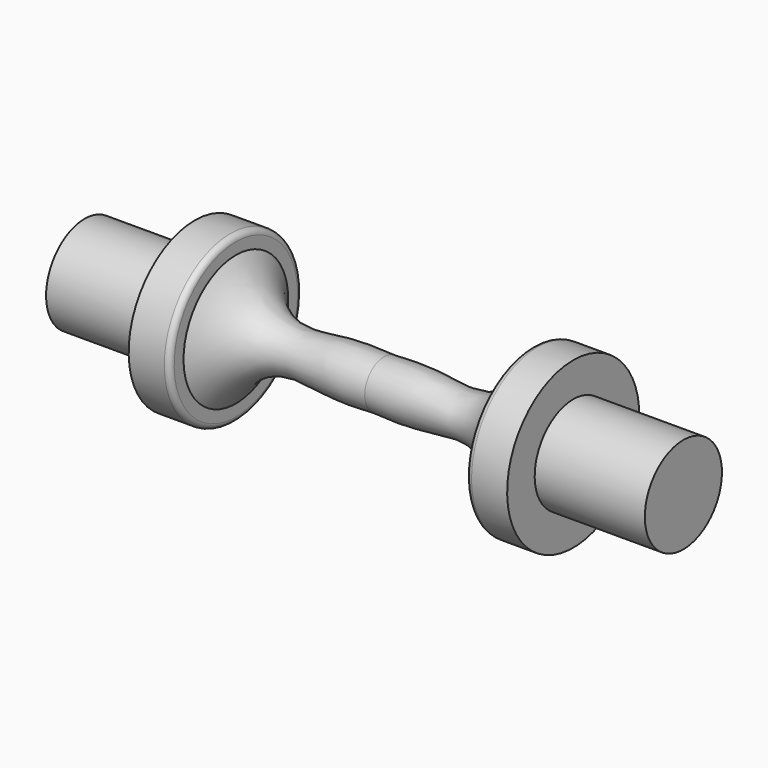
from build123d import *


with BuildPart() as f1:
    # F0 (on Front) → F1 (revolve)
    with BuildSketch(Plane.XZ):
        with BuildLine():
            Line((0, 8.75), (0, 0))
            Line((0, 0), (108.719505762, 0))
            Line((108.719505762, 0), (108.719505762, 17.5))
            Line((108.719505762, 17.5), (68.719505762, 17.5))
            Line((68.719505762, 17.5), (68.719505762, 30))
            Line((68.719505762, 30), (55.7926830174, 30))
            ThreePointArc((55.7926830174, 30), (54.3784694551, 29.4142135624), (53.7926830174, 28))
            Line((53.7926830174, 28), (53.7926830174, 23.75))
            add(Edge.make_bspline(
                [(0, 8.75), (5.0406153604, 9.0258980354), (16.3424850669, 9.5343195461), (38.0075656916, 5.0292358393), (49.6364947054, 17.2036020787), (53.7926830174, 23.75)],
                knots=[0, 0, 0, 0, 0.3026453885, 0.6427893554, 1, 1, 1, 1], degree=3))
        make_face()
    revolve(axis=Axis((54.359752881, 0, 0), (-1, 0, 0)))

    # F2: F1 across face


with BuildPart() as f1_1:
    add(f1.part)
    add(f1.part.mirror(Plane(origin=(0, 0, 0), x_dir=(0, -1, 0), z_dir=(-1, 0, 0))))


solid = f1_1.part
